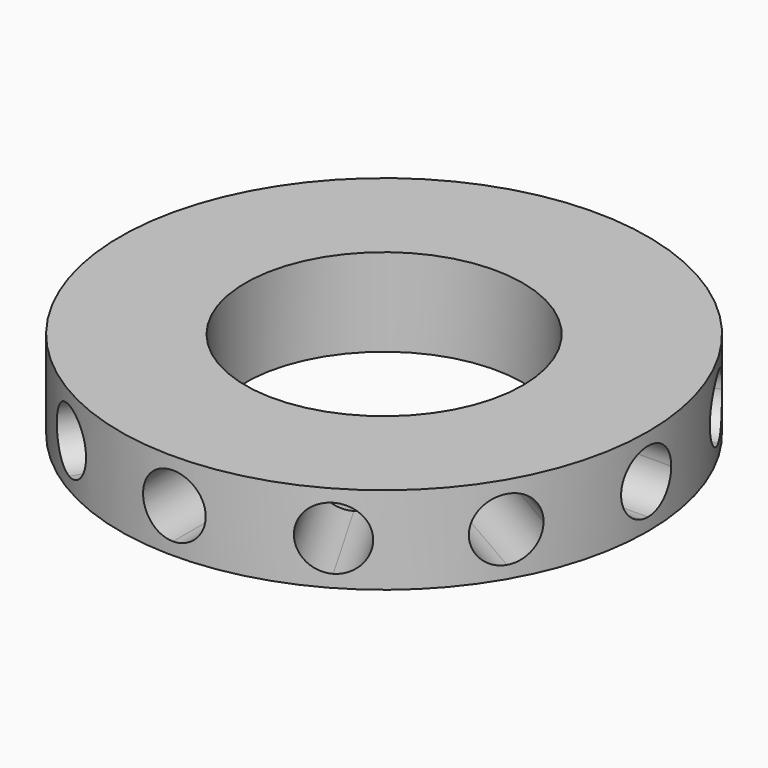
from build123d import *

# Parameters (mm, degrees)
F0_R            = 21.075
F0_R_2          = 11.075
F1_DEPTH        = 7
F4_DEPTH        = 12.5
F4_COPIES_COUNT = 12


# Not quite as in the source:
# - a pattern or mirror of a feature is missing from the dataset's text; its kind, count and spacing are read off the source's solid


with BuildPart() as f1:
    # F0 (on Top) → F1 (new body)
    with BuildSketch(Plane.XY):
        Circle(F0_R)
        Circle(F0_R_2, mode=Mode.SUBTRACT)
    extrude(amount=F1_DEPTH)

    # F3 (on offset) → F4 (cut)
    with BuildSketch(Plane.XZ.offset(25)):
        with BuildLine():
            Line((0, 1), (0, 6))
            ThreePointArc((0, 6), (-2.5, 3.5), (0, 1))
        make_face()
        with BuildLine():
            ThreePointArc((0, 1), (1.767766953, 1.732233047), (2.5, 3.5))
            ThreePointArc((2.5, 3.5), (1.767766953, 5.267766953), (0, 6))
            Line((0, 6), (0, 1))
        make_face()
    f4 = extrude(amount=-F4_DEPTH, mode=Mode.SUBTRACT)

    # F4_copies: F4 ×12 about axis
    f4_copies_axis = Axis((0, 0, 0), (0, 0, 1))
    for i in range(1, F4_COPIES_COUNT):
        add(f4.rotate(f4_copies_axis, i * 360 / F4_COPIES_COUNT), mode=Mode.SUBTRACT)


solid = f1.part
